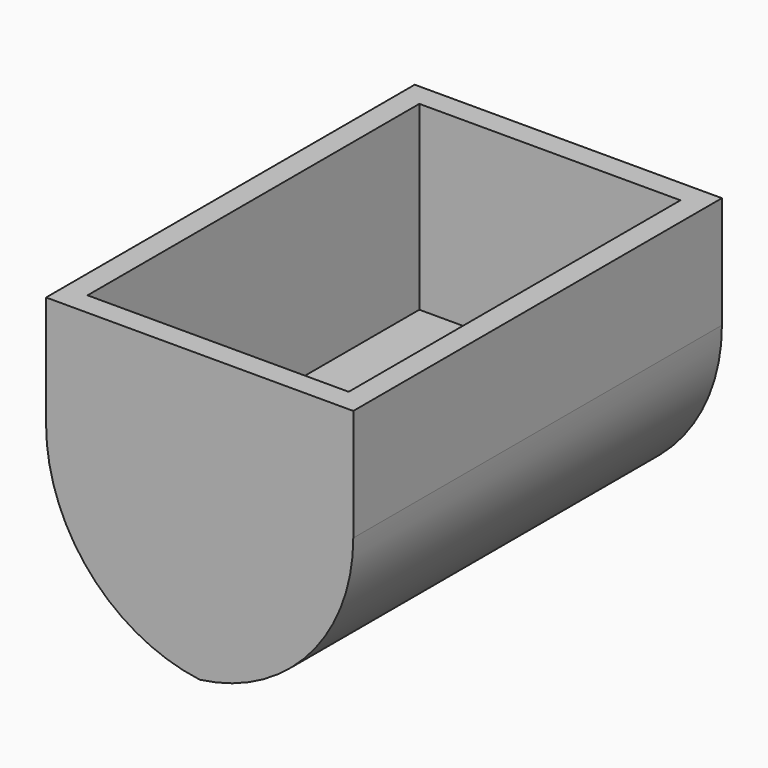
from build123d import *

# Parameters (mm, degrees)
F0_W        = 101.6
F0_H        = 152.4
F1_DEPTH    = 95.25
F2_T1_DEPTH = 443.6748663003
F4_DEPTH    = 59.944


# Not quite as in the source:
# - a fillet or chamfer that OpenCascade refuses, or shapes differently, is made with other operations: its cross-section is extruded or revolved along the edge and cut away or added


with BuildPart() as f1:
    # F0 (on Top) → F1 (new body)
    with BuildSketch(Plane.XY):
        with Locations((2.2735033583, 3.7213955075)):
            Rectangle(F0_W, F0_H)
    extrude(amount=F1_DEPTH)

    # F2: fillet of radius 58.2549732601 on 2 edges, made by hand

    # F2_s2 → F2_t1 (cut)
    with BuildSketch(Plane.XZ.offset(-225.5588286576)):
        with BuildLine():
            ThreePointArc((-48.5264966417, 58.2549732601), (-31.4640100116, 17.06248663), (9.7284766184, 0))
            Line((9.7284766184, 0), (-48.5264966417, 0))
            Line((-48.5264966417, 0), (-48.5264966417, 58.2549732601))
        make_face()
        with BuildLine():
            ThreePointArc((53.0735033583, 58.2549732601), (36.0110167283, 17.06248663), (-5.1814699017, 0))
            Line((-5.1814699017, 0), (53.0735033583, 0))
            Line((53.0735033583, 0), (53.0735033583, 58.2549732601))
        make_face()
    extrude(amount=F2_T1_DEPTH, mode=Mode.SUBTRACT)

    # F3 (on face) → F4 (cut)
    with BuildSketch(Plane.XY.offset(95.25)):
        Polygon((-40.9064966417, 17.4030140042), (-40.9064966417, -64.8586044925), (45.4535033583, -64.8586044925), (45.4535033583, 17.9895181209), (45.4535033583, 72.3013955075), (-40.9064966417, 72.3013955075), align=None)
    extrude(amount=-F4_DEPTH, mode=Mode.SUBTRACT)


solid = f1.part
